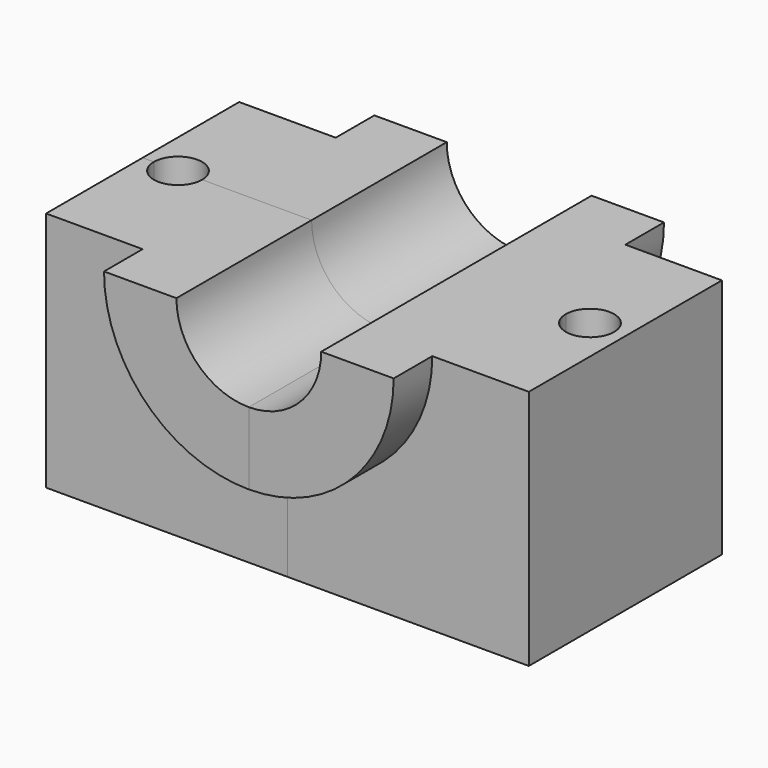
from build123d import *
from build123d import SkipClean  # not in build123d's __all__

# Parameters (mm, degrees)
F1_DEPTH = 100
F3_DEPTH = 20
F4_DEPTH = 50


with BuildPart() as f1:
    # F0 (on Top) → F1 (new body)
    with BuildSketch(Plane.XY):
        with BuildLine():
            Line((-100, -50), (0, -50))
            Line((0, -50), (0, 0))
            Line((0, 0), (-75.3427499533, 0))
            ThreePointArc((-75.3427499533, 0), (-85.3427499533, -10), (-95.3427499533, 0))
            Line((-95.3427499533, 0), (-100, 0))
            Line((-100, 0), (-100, -50))
        make_face()
    extrude(amount=F1_DEPTH)

    # F2 (on face) → F3 (join)
    with BuildSketch(Plane.XZ.offset(50)):
        with BuildLine():
            ThreePointArc((0, 70), (-21.2132034356, 78.7867965644), (-30, 100))
            Line((-30, 100), (-60, 100))
            ThreePointArc((-60, 100), (-42.4264068712, 57.5735931288), (0, 40))
            Line((0, 40), (0, 70))
        make_face()
    extrude(amount=F3_DEPTH)

    # F4 (cut, through all): a face of the model
    f4_faces = [f1.faces().sort_by_distance(p)[0] for p in [
        (-12.7323954474, -50, 87.2676045526),
    ]]
    extrude(f4_faces, amount=-F4_DEPTH, mode=Mode.SUBTRACT)

    # F5: F1 across plane


with BuildPart() as f1_1:
    add(f1.part, clean=False)
    with SkipClean():  # cleaning this boolean's faces spoils the solid; the shape is the same uncleaned
        add(f1.part.mirror(Plane.XZ), clean=False)

    # F6: F1 across face


with BuildPart() as f1_2:
    add(f1_1.part, clean=False)
    add(f1_1.part.mirror(Plane(origin=(0, -30.1219512195, 37.9268292683), x_dir=(0, 1, 0), z_dir=(1, 0, 0))), clean=False)


solid = f1_2.part
